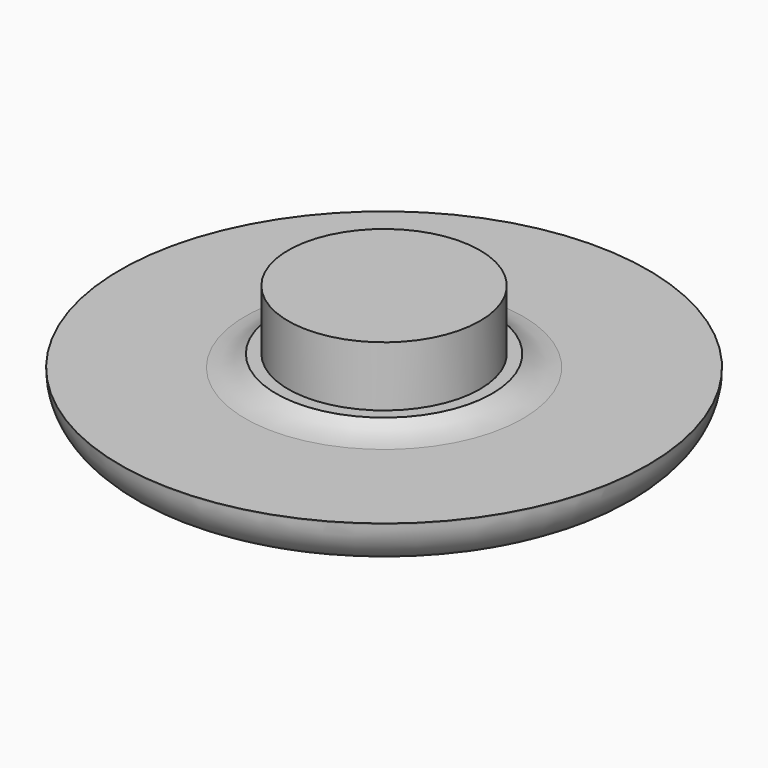
from build123d import *

# Parameters (mm, degrees)
F0_R     = 11
F1_DEPTH = 2
F2_R     = 4.5
F3_DEPTH = 0.5
F4_R     = 3.995
F5_DEPTH = 2.5


# Not quite as in the source:
# - a fillet or chamfer that OpenCascade refuses, or shapes differently, is made with other operations: its cross-section is extruded or revolved along the edge and cut away or added


with BuildPart() as f1:
    # F0 (on Top) → F1 (new body)
    with BuildSketch(Plane.XY):
        with Locations((-124.7583553195, 13.61318212)):
            Circle(F0_R)
    extrude(amount=F1_DEPTH)

    # F2 (on face) → F3 (join)
    with BuildSketch(Plane.XY.offset(2)):
        with Locations((-124.7583553195, 13.61318212)):
            Circle(F2_R)
    extrude(amount=F3_DEPTH)

    # F4 (on face) → F5 (join)
    with BuildSketch(Plane.XY.offset(2.5)):
        with Locations((-124.7583553195, 13.61318212)):
            Circle(F4_R)
    extrude(amount=F5_DEPTH)

    # F6: fillet of radius 2 on 2 edges, made by hand

    # F6_s1 → F6_t2 (revolve)
    with BuildSketch(Plane.XZ.offset(-13.61318212)):
        with BuildLine():
            ThreePointArc((-118.9351147195, 1.9996), (-119.642533578, 2.1287949759), (-120.2586198399, 2.4996999517))
            Line((-120.2586198399, 2.4996999517), (-120.3909703519, 2.3495733784))
            ThreePointArc((-120.3909703519, 2.3495733784), (-120.458491888, 2.2498499759), (-120.458491888, 2))
            Line((-120.458491888, 2), (-120.2583553195, 1.7998634315))
            ThreePointArc((-120.2583553195, 1.7998634315), (-119.5967350195, 1.7998634315), (-118.9351147195, 1.7994634315))
            Line((-118.9351147195, 1.7994634315), (-118.9351147195, 1.9996))
        make_face()
    revolve(axis=Axis((-124.7583553195, 13.61318212, 2), (0, 0, 1)))

    # F6_s3 → F6_t4 (revolve, cut)
    with BuildSketch(Plane.XZ.offset(-13.61318212)):
        with BuildLine():
            ThreePointArc((-113.7579553195, 1.999999807), (-114.3444830549, 0.5854449892), (-115.7593207719, -0.0004))
            Line((-115.7593207719, -0.0004), (-115.7593207719, -0.2005365685))
            ThreePointArc((-115.7593207719, -0.2005365685), (-114.7588380457, -0.2001365685), (-113.7583553195, -0.2001365685))
            Line((-113.7583553195, -0.2001365685), (-113.558218751, 0))
            ThreePointArc((-113.558218751, 0), (-113.558218751, 0.9999999035), (-113.5578187743, 1.9999032191))
            Line((-113.5578187743, 1.9999032191), (-113.7579553195, 1.999999807))
        make_face()
    revolve(axis=Axis((-124.7583553195, 13.61318212, 0), (0, 0, 1)), mode=Mode.SUBTRACT)


solid = f1.part
